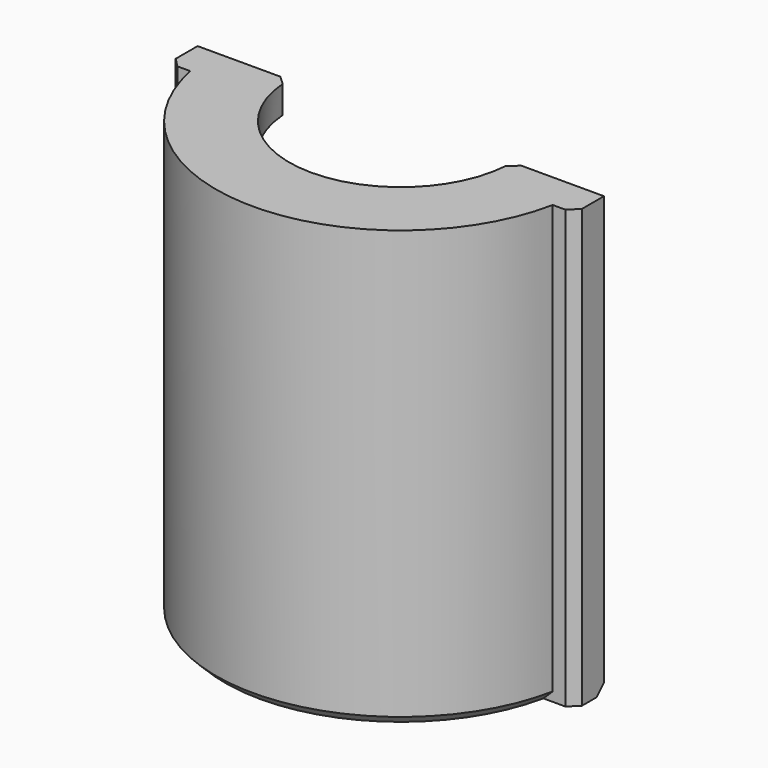
from build123d import *
from build123d import SkipClean  # not in build123d's __all__

# Parameters (mm, degrees)
F0_W         = 2
F0_H         = 1.2
F1_ANGLE     = 180
F3_DEPTH     = 29
F5_DEPTH     = 30.5
F6_DEPTH     = 6.6
F7_T1_DEPTH  = 26.471682988
F7_T3_DEPTH  = 14.2
F7_T5_DEPTH  = 2.285841494
F7_T7_DEPTH  = 3.285841494
F7_T9_DEPTH  = 3.9794390696
F7_T11_DEPTH = 3.285841494
F7_T13_DEPTH = 2.285841494
F7_T15_DEPTH = 2.4504714643
F7_T17_DEPTH = 1.2
F7_T19_DEPTH = 5.8
F7_T24_ANGLE = 171.7642778101
F8_T1_DEPTH  = 2.5339152929
F8_T3_DEPTH  = 2.7820723675
F8_T5_DEPTH  = 2.7820723675
F8_T7_DEPTH  = 2.5339152929
F8_T10_ANGLE = 70.8970289143
F8_T12_ANGLE = 70.8970289143
F8_T14_ANGLE = 70.8970289143
F8_T16_ANGLE = 70.8970289143
F8_T18_ANGLE = 70.8970289143
F8_T20_ANGLE = 70.8970289143
F8_T22_ANGLE = 70.8970289143
F8_T24_ANGLE = 70.8970289143


# Not quite as in the source:
# - a fillet or chamfer that OpenCascade refuses, or shapes differently, is made with other operations: its cross-section is extruded or revolved along the edge and cut away or added
# - a feature names something its author has since deleted; it is built from what else it names


with BuildPart() as f1:
    # F0 (on Front) → F1 (revolve)
    with BuildSketch(Plane.XZ):
        Polygon((-10.1, 0), (-8.1, 0), (-8.1, 6.6), (-8.1, 7.8), (-8.1, 12.7), (-8.1, 13.9), (-8.1, 15.8), (-8.1, 17), (-8.1, 22), (-8.1, 23.2), (-8.1, 29), (-10.1, 29), align=None)
        with Locations((-7.1, 22.6)):
            Rectangle(F0_W, F0_H)
        with Locations((-7.1, 7.2)):
            Rectangle(F0_W, F0_H)
        Polygon((-10.1, 30.5), (-10.1, 29), (-8.1, 29), (-6.1, 29), (-6.1, 30.5), align=None)
    revolve(axis=Axis((0, 0, 18.970021978), (0, 0, 1)), revolution_arc=F1_ANGLE)

    # F2 (on face) → F3 (cut, through all)
    with BuildSketch(Plane(origin=(0, 0, 0), x_dir=(1, 0, 0), z_dir=(0, 0, -1))):
        with BuildLine():
            Line((2.5, 5.5641710973), (2.5, 7.7045441137))
            ThreePointArc((2.5, 7.7045441137), (0, 8.1), (-2.5, 7.7045441137))
            Line((-2.5, 7.7045441137), (-2.5, 5.5641710973))
            Line((-2.5, 5.5641710973), (2.5, 5.5641710973))
        make_face()
        with BuildLine():
            ThreePointArc((8.1, 0), (8.0648988191, 0.7532642549), (7.9598994969, 1.5))
            Line((7.9598994969, 1.5), (5.9126981996, 1.5))
            Line((5.9126981996, 1.5), (5.9126981996, 0))
            Line((5.9126981996, 0), (8.1, 0))
        make_face()
        with BuildLine():
            Line((-5.9126981996, 1.5), (-7.9598994969, 1.5))
            ThreePointArc((-7.9598994969, 1.5), (-8.0648988191, 0.7532642549), (-8.1, 0))
            Line((-8.1, 0), (-5.9126981996, 0))
            Line((-5.9126981996, 0), (-5.9126981996, 1.5))
        make_face()
    with SkipClean():  # cleaning this boolean's faces spoils the solid; the shape is the same uncleaned
        extrude(amount=-F3_DEPTH, mode=Mode.SUBTRACT)

    # F4 (on face) → F5 (join, through all)
    with BuildSketch(Plane(origin=(0, 0, 0), x_dir=(1, 0, 0), z_dir=(0, 0, -1))):
        with BuildLine():
            Line((11.1, 2), (9.9, 2))
            ThreePointArc((9.9, 2), (10.0498756211, 1.0049875621), (10.1, 0))
            Line((10.1, 0), (11.1, 0))
            Line((11.1, 0), (11.1, 2))
        make_face()
        with BuildLine():
            Line((-11.1, 0), (-10.1, 0))
            ThreePointArc((-10.1, 0), (-10.0498756211, 1.0049875621), (-9.9, 2))
            Line((-9.9, 2), (-11.1, 2))
            Line((-11.1, 2), (-11.1, 0))
        make_face()
    with SkipClean():  # cleaning this boolean's faces spoils the solid; the shape is the same uncleaned
        extrude(amount=-F5_DEPTH)

    # F4 (on face) + F2 (on face) → F6 (cut, through all)
    with BuildSketch(Plane(origin=(0, 0, 0), x_dir=(1, 0, 0), z_dir=(0, 0, -1))):
        with BuildLine():
            Line((-9.1, 2), (-9.1, 0))
            Line((-9.1, 0), (-8.1, 0))
            ThreePointArc((-8.1, 0), (-8.0648988191, 0.7532642549), (-7.9598994969, 1.5))
            ThreePointArc((-7.9598994969, 1.5), (-6.0808277632, 5.3510310889), (-2.5, 7.7045441137))
            ThreePointArc((-2.5, 7.7045441137), (0, 8.1), (2.5, 7.7045441137))
            ThreePointArc((2.5, 7.7045441137), (6.0808277632, 5.3510310889), (7.9598994969, 1.5))
            ThreePointArc((7.9598994969, 1.5), (8.0648988191, 0.7532642549), (8.1, 0))
            Line((8.1, 0), (9.1, 0))
            Line((9.1, 0), (9.1, 2))
            Line((9.1, 2), (9.9, 2))
            ThreePointArc((9.9, 2), (0, 10.1), (-9.9, 2))
            Line((-9.9, 2), (-9.1, 2))
        make_face()
        with BuildLine():
            Line((-11.1, 0), (-10.1, 0))
            ThreePointArc((-10.1, 0), (-10.0498756211, 1.0049875621), (-9.9, 2))
            Line((-9.9, 2), (-11.1, 2))
            Line((-11.1, 2), (-11.1, 0))
        make_face()
        with BuildLine():
            Line((-10.1, 0), (-9.1, 0))
            Line((-9.1, 0), (-9.1, 2))
            Line((-9.1, 2), (-9.9, 2))
            ThreePointArc((-9.9, 2), (-10.0498756211, 1.0049875621), (-10.1, 0))
        make_face()
        with BuildLine():
            Line((11.1, 2), (9.9, 2))
            ThreePointArc((9.9, 2), (10.0498756211, 1.0049875621), (10.1, 0))
            Line((10.1, 0), (11.1, 0))
            Line((11.1, 0), (11.1, 2))
        make_face()
    with BuildSketch(Plane(origin=(0, 0, 0), x_dir=(1, 0, 0), z_dir=(0, 0, -1))):
        with BuildLine():
            ThreePointArc((-2.5, 7.7045441137), (0, 8.1), (2.5, 7.7045441137))
            ThreePointArc((2.5, 7.7045441137), (6.0808277632, 5.3510310889), (7.9598994969, 1.5))
            ThreePointArc((7.9598994969, 1.5), (8.0648988191, 0.7532642549), (8.1, 0))
            Line((8.1, 0), (10.1, 0))
            ThreePointArc((10.1, 0), (0, 10.1), (-10.1, 0))
            Line((-10.1, 0), (-8.1, 0))
            ThreePointArc((-8.1, 0), (-8.0648988191, 0.7532642549), (-7.9598994969, 1.5))
            ThreePointArc((-7.9598994969, 1.5), (-6.0808277632, 5.3510310889), (-2.5, 7.7045441137))
        make_face()
    with SkipClean():  # cleaning this boolean's faces spoils the solid; the shape is the same uncleaned
        extrude(amount=-F6_DEPTH, mode=Mode.SUBTRACT)

    # F7: chamfer of 0.5 on 11 edges, made by hand

    # F7_s2 → F7_t1 (cut)
    with BuildSketch(Plane.XY.offset(5.314158506)):
        Polygon((-10.6, -2), (-11.1, -1.5), (-11.1, -2), align=None)
        Polygon((10.6, -2), (11.1, -1.5), (11.1, -2), align=None)
    with SkipClean():  # cleaning this boolean's faces spoils the solid; the shape is the same uncleaned
        extrude(amount=F7_T1_DEPTH, mode=Mode.SUBTRACT)

    # F7_s4 → F7_t3 (cut)
    with BuildSketch(Plane.XY.offset(7.8)):
        with BuildLine():
            Line((8.5854528128, 0), (8.0862985795, -0.4709302326))
            ThreePointArc((8.0862985795, -0.4709302326), (8.0963649191, -0.2426419097), (8.1, 0))
            Line((8.1, 0), (8.5854528128, 0))
        make_face()
        with BuildLine():
            Line((-8.5854528128, 0), (-8.0862985795, -0.4709302326))
            ThreePointArc((-8.0862985795, -0.4709302326), (-8.0963649191, -0.2426419097), (-8.1, 0))
            Line((-8.1, 0), (-8.5854528128, 0))
        make_face()
    extrude(amount=F7_T3_DEPTH, mode=Mode.SUBTRACT)

    # F7_s6 → F7_t5 (cut)
    with BuildSketch(Plane.YZ.offset(-12.385841494)):
        Polygon((-0.5, 6.6), (0, 7.1), (0, 6.6), align=None)
    extrude(amount=F7_T5_DEPTH, mode=Mode.SUBTRACT)

    # F7_s8 → F7_t7 (cut)
    with BuildSketch(Plane.YZ.offset(-10.1)):
        Polygon((-0.5, 6.6), (0, 7.1), (0, 6.6), align=None)
    extrude(amount=F7_T7_DEPTH, mode=Mode.SUBTRACT)

    # F7_s10 → F7_t9 (cut)
    with BuildSketch(Plane.XY.offset(27.7602804652)):
        with BuildLine():
            Line((-6.5810333535, 0), (-6.0824702207, -0.4621212121))
            ThreePointArc((-6.0824702207, -0.4621212121), (-6.0953433287, -0.2383059061), (-6.1, 0))
            Line((-6.1, 0), (-6.5810333535, 0))
        make_face()
        with BuildLine():
            Line((6.5810333535, 0), (6.0824702207, -0.4621212121))
            ThreePointArc((6.0824702207, -0.4621212121), (6.0953433287, -0.2383059061), (6.1, 0))
            Line((6.1, 0), (6.5810333535, 0))
        make_face()
    with SkipClean():  # cleaning this boolean's faces spoils the solid; the shape is the same uncleaned
        extrude(amount=F7_T9_DEPTH, mode=Mode.SUBTRACT)

    # F7_s12 → F7_t11 (cut)
    with BuildSketch(Plane.YZ.offset(6.814158506)):
        Polygon((-0.5, 6.6), (0, 7.1), (0, 6.6), align=None)
    extrude(amount=F7_T11_DEPTH, mode=Mode.SUBTRACT)

    # F7_s14 → F7_t13 (cut)
    with BuildSketch(Plane.YZ.offset(10.1)):
        Polygon((-0.5, 6.6), (0, 7.1), (0, 6.6), align=None)
    extrude(amount=F7_T13_DEPTH, mode=Mode.SUBTRACT)

    # F7_s16 → F7_t15 (cut)
    with BuildSketch(Plane.XY.offset(5.3495285357)):
        with BuildLine():
            Line((-8.0862985795, -0.4709302326), (-8.5854528128, 0))
            Line((-8.5854528128, 0), (-8.1, 0))
            ThreePointArc((-8.1, 0), (-8.0963649191, -0.2426419097), (-8.0862985795, -0.4709302326))
        make_face()
        with BuildLine():
            Line((8.0862985795, -0.4709302326), (8.5854528128, 0))
            Line((8.5854528128, 0), (8.1, 0))
            ThreePointArc((8.1, 0), (8.0963649191, -0.2426419097), (8.0862985795, -0.4709302326))
        make_face()
    with SkipClean():  # cleaning this boolean's faces spoils the solid; the shape is the same uncleaned
        extrude(amount=F7_T15_DEPTH, mode=Mode.SUBTRACT)

    # F7_s18 → F7_t17 (cut)
    with BuildSketch(Plane.XY.offset(22)):
        with BuildLine():
            Line((-8.5854528128, 0), (-8.0862985795, -0.4709302326))
            ThreePointArc((-8.0862985795, -0.4709302326), (-8.0963649191, -0.2426419097), (-8.1, 0))
            Line((-8.1, 0), (-8.5854528128, 0))
        make_face()
        with BuildLine():
            Line((8.5854528128, 0), (8.0862985795, -0.4709302326))
            ThreePointArc((8.0862985795, -0.4709302326), (8.0963649191, -0.2426419097), (8.1, 0))
            Line((8.1, 0), (8.5854528128, 0))
        make_face()
    with SkipClean():  # cleaning this boolean's faces spoils the solid; the shape is the same uncleaned
        extrude(amount=F7_T17_DEPTH, mode=Mode.SUBTRACT)

    # F7_s20 → F7_t19 (cut)
    with BuildSketch(Plane.XY.offset(23.2)):
        with BuildLine():
            Line((-8.5854528128, 0), (-8.0862985795, -0.4709302326))
            ThreePointArc((-8.0862985795, -0.4709302326), (-8.0963649191, -0.2426419097), (-8.1, 0))
            Line((-8.1, 0), (-8.5854528128, 0))
        make_face()
        with BuildLine():
            Line((8.5854528128, 0), (8.0862985795, -0.4709302326))
            ThreePointArc((8.0862985795, -0.4709302326), (8.0963649191, -0.2426419097), (8.1, 0))
            Line((8.1, 0), (8.5854528128, 0))
        make_face()
    with SkipClean():  # cleaning this boolean's faces spoils the solid; the shape is the same uncleaned
        extrude(amount=F7_T19_DEPTH, mode=Mode.SUBTRACT)


with BuildPart() as f7_tool22:
    # F7_s23 → F7_t24 (revolve)
    with BuildSketch(Plane(origin=(0, 0, 0), x_dir=(0, 0, 1), z_dir=(0.071808378, 0.9974184462, 0))):
        Polygon((7.1, 10.1), (6.6, 9.6), (6.6, 10.1), align=None)
    revolve(axis=Axis((0, 0, 6.6), (0, 0, -1)), revolution_arc=F7_T24_ANGLE)

    split(bisect_by=Plane.XZ.offset(2), keep=Keep.TOP)


with BuildPart() as f1_1:
    add(f1.part, clean=False)

    # F7_t21: cut F7_tool22
    add(f7_tool22.part, mode=Mode.SUBTRACT)

    # F8: chamfer of 0.4 on 16 edges, made by hand

    # F8_s2 → F8_t1 (cut)
    with BuildSketch(Plane.XY.offset(5.9330423536)):
        with BuildLine():
            Line((2.7215384615, -5.4592333164), (2.5, -5.8172158289))
            Line((2.5, -5.8172158289), (2.5, -5.5641710973))
            ThreePointArc((2.5, -5.5641710973), (2.6173705778, -5.5099338706), (2.7215384615, -5.4592333164))
        make_face()
        with BuildLine():
            Line((-2.5, -5.8172158289), (-2.7215384615, -5.4592333164))
            ThreePointArc((-2.7215384615, -5.4592333164), (-2.6173705778, -5.5099338706), (-2.5, -5.5641710973))
            Line((-2.5, -5.5641710973), (-2.5, -5.8172158289))
        make_face()
    extrude(amount=F8_T1_DEPTH, mode=Mode.SUBTRACT)

    # F8_s4 → F8_t3 (cut)
    with BuildSketch(Plane.XY.offset(5.8089638162)):
        with BuildLine():
            Line((6.2161081072, -1.5), (5.8335783775, -1.7830769231))
            ThreePointArc((5.8335783775, -1.7830769231), (5.8731388435, -1.6481019766), (5.9126981996, -1.5))
            Line((5.9126981996, -1.5), (6.2161081072, -1.5))
        make_face()
        with BuildLine():
            Line((-5.8335783775, -1.7830769231), (-6.2161081072, -1.5))
            Line((-6.2161081072, -1.5), (-5.9126981996, -1.5))
            ThreePointArc((-5.9126981996, -1.5), (-5.8731388435, -1.6481019766), (-5.8335783775, -1.7830769231))
        make_face()
    extrude(amount=F8_T3_DEPTH, mode=Mode.SUBTRACT)

    # F8_s6 → F8_t5 (cut)
    with BuildSketch(Plane.XY.offset(21.2089638162)):
        with BuildLine():
            Line((-6.2161081072, -1.5), (-5.8335783775, -1.7830769231))
            ThreePointArc((-5.8335783775, -1.7830769231), (-5.8731388435, -1.6481019766), (-5.9126981996, -1.5))
            Line((-5.9126981996, -1.5), (-6.2161081072, -1.5))
        make_face()
        with BuildLine():
            Line((5.8335783775, -1.7830769231), (6.2161081072, -1.5))
            Line((6.2161081072, -1.5), (5.9126981996, -1.5))
            ThreePointArc((5.9126981996, -1.5), (5.8731388435, -1.6481019766), (5.8335783775, -1.7830769231))
        make_face()
    extrude(amount=F8_T5_DEPTH, mode=Mode.SUBTRACT)

    # F8_s8 → F8_t7 (cut)
    with BuildSketch(Plane.XY.offset(21.3330423536)):
        with BuildLine():
            Line((-2.5, -5.8172158289), (-2.7215384615, -5.4592333164))
            ThreePointArc((-2.7215384615, -5.4592333164), (-2.6173705778, -5.5099338706), (-2.5, -5.5641710973))
            Line((-2.5, -5.5641710973), (-2.5, -5.8172158289))
        make_face()
        with BuildLine():
            Line((2.7215384615, -5.4592333164), (2.5, -5.8172158289))
            Line((2.5, -5.8172158289), (2.5, -5.5641710973))
            ThreePointArc((2.5, -5.5641710973), (2.6173705778, -5.5099338706), (2.7215384615, -5.4592333164))
        make_face()
    extrude(amount=F8_T7_DEPTH, mode=Mode.SUBTRACT)

    # F8_s9 → F8_t10 (revolve, cut)
    with BuildSketch(Plane(origin=(0, 0, 0), x_dir=(0, 0, 1), z_dir=(-0.968011189, -0.2509070307, 0))):
        Polygon((7.8, -6.5), (7.4, -6.1), (7.8, -6.1), align=None)
    revolve(axis=Axis((0, 0, 7.8), (0, 0, 1)), revolution_arc=F8_T10_ANGLE, mode=Mode.SUBTRACT)

    # F8_s11 → F8_t12 (revolve, cut)
    with BuildSketch(Plane(origin=(0, 0, 0), x_dir=(0, 0, 1), z_dir=(-0.968011189, -0.2509070307, 0))):
        Polygon((6.6, -6.5), (7, -6.1), (6.6, -6.1), align=None)
    revolve(axis=Axis((0, 0, 6.6), (0, 0, 1)), revolution_arc=F8_T12_ANGLE, mode=Mode.SUBTRACT)

    # F8_s13 → F8_t14 (revolve, cut)
    with BuildSketch(Plane(origin=(0, 0, 0), x_dir=(0, 0, 1), z_dir=(-0.0797079521, 0.9968182594, 0))):
        Polygon((7.8, -6.5), (7.4, -6.1), (7.8, -6.1), align=None)
    revolve(axis=Axis((0, 0, 7.8), (0, 0, 1)), revolution_arc=F8_T14_ANGLE, mode=Mode.SUBTRACT)

    # F8_s15 → F8_t16 (revolve, cut)
    with BuildSketch(Plane(origin=(0, 0, 0), x_dir=(0, 0, 1), z_dir=(-0.0797079521, 0.9968182594, 0))):
        Polygon((6.6, -6.5), (7, -6.1), (6.6, -6.1), align=None)
    revolve(axis=Axis((0, 0, 6.6), (0, 0, 1)), revolution_arc=F8_T16_ANGLE, mode=Mode.SUBTRACT)

    # F8_s17 → F8_t18 (revolve, cut)
    with BuildSketch(Plane(origin=(0, 0, 0), x_dir=(0, 0, 1), z_dir=(-0.0797079521, 0.9968182594, 0))):
        Polygon((23.2, -6.5), (22.8, -6.1), (23.2, -6.1), align=None)
    revolve(axis=Axis((0, 0, 23.2), (0, 0, 1)), revolution_arc=F8_T18_ANGLE, mode=Mode.SUBTRACT)

    # F8_s19 → F8_t20 (revolve, cut)
    with BuildSketch(Plane(origin=(0, 0, 0), x_dir=(0, 0, 1), z_dir=(-0.0797079521, 0.9968182594, 0))):
        Polygon((22.4, -6.1), (22, -6.5), (22, -6.1), align=None)
    revolve(axis=Axis((0, 0, 22), (0, 0, 1)), revolution_arc=F8_T20_ANGLE, mode=Mode.SUBTRACT)

    # F8_s21 → F8_t22 (revolve, cut)
    with BuildSketch(Plane(origin=(0, 0, 0), x_dir=(0, 0, 1), z_dir=(-0.968011189, -0.2509070307, 0))):
        Polygon((23.2, -6.5), (22.8, -6.1), (23.2, -6.1), align=None)
    revolve(axis=Axis((0, 0, 23.2), (0, 0, 1)), revolution_arc=F8_T22_ANGLE, mode=Mode.SUBTRACT)

    # F8_s23 → F8_t24 (revolve, cut)
    with BuildSketch(Plane(origin=(0, 0, 0), x_dir=(0, 0, 1), z_dir=(-0.968011189, -0.2509070307, 0))):
        Polygon((22.4, -6.1), (22, -6.5), (22, -6.1), align=None)
    revolve(axis=Axis((0, 0, 22), (0, 0, 1)), revolution_arc=F8_T24_ANGLE, mode=Mode.SUBTRACT)


solid = f1_1.part
